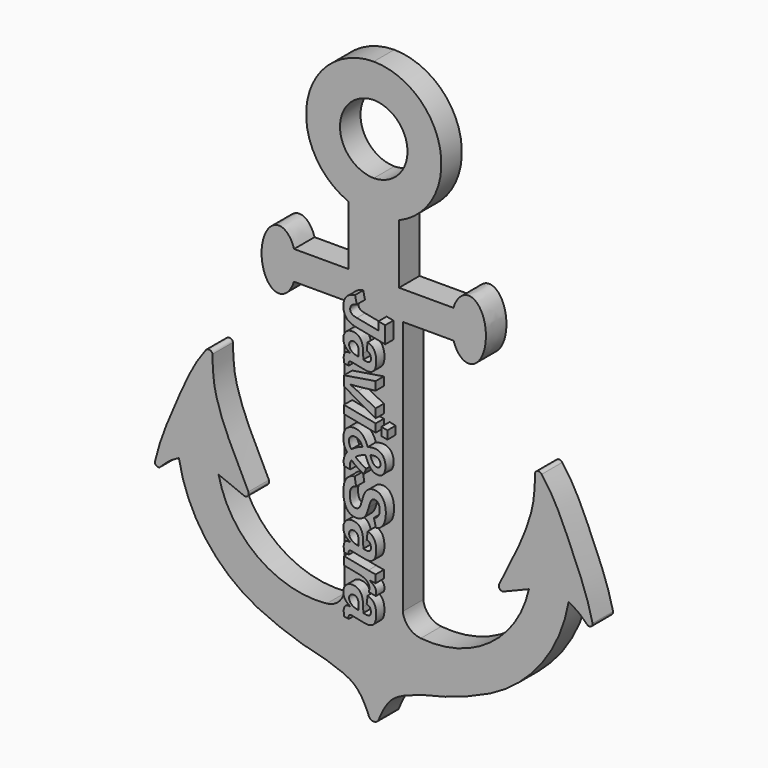
from build123d import *

# Parameters (mm, degrees)
F1_DEPTH     = 2.5
F2_TEXT_SIZE = 5.843307762
F3_DEPTH     = 1


# Not quite as in the source:
# - Text() gives the source's letters only with a copy of the font that has no kerning and outlines rounded to 1/6400 em; it was checked with that copy


with BuildPart() as f1:
    # F0 (on Front) → F1 (new body)
    with BuildSketch(Plane.XZ):
        Polygon((19.9702170016, 32.0593795983), (15.0368500231, 32.0593795983), (15.0368500231, 26.2546902991), (9.737966444, 26.2546902991), (9.7163520504, 23.4430860728), (14.649162069, 23.4430860728), (14.649162069, -1.4119866537), (14.6655309945, -1.4119866537), (20.3415360302, -1.4119866537), (20.3579049557, -1.4119866537), (20.3579049557, 23.4430860728), (25.2907149743, 23.4430860728), (25.2767818304, 26.2546902991), (25.2691005807, 26.2546902991), (19.9702170016, 26.2546902991), align=None)
        with BuildLine():
            add(Edge.make_bspline(
                [(25.2907149743, 23.4430860728), (26.2882305831, 20.365262945), (27.8484616427, 22.637675937), (29.4086927023, 24.9100889291), (27.8261704411, 27.1358736943), (26.2436481799, 29.3616584594), (25.2767818304, 26.2546902991)],
                knots=[2.0818835057, 2.0818835057, 2.0818835057, 3.8412701203, 3.8412701203, 5.6006567348, 5.6006567348, 7.3600433494, 7.3600433494, 7.3600433494], degree=2, weights=[1, 0.6373874942, 1, 0.6373874942, 1, 0.6373874942, 1]))
            Line((25.2767818304, 26.2546902991), (25.2907149743, 23.4430860728))
        make_face()
        with BuildLine():
            ThreePointArc((19.9702170016, 32.0593795983), (23.9805343506, 39.4793828594), (17.5035335124, 44.8819335324))
            ThreePointArc((17.5035335124, 44.8819335324), (11.0265326741, 39.4793828594), (15.0368500231, 32.0593795983))
            Line((15.0368500231, 32.0593795983), (19.9702170016, 32.0593795983))
        make_face()
        with BuildLine():
            ThreePointArc((17.5035335124, 34.864031021), (14.2101902268, 38.22103329), (17.5035335124, 41.578035559))
            ThreePointArc((17.5035335124, 41.578035559), (20.796876798, 38.22103329), (17.5035335124, 34.864031021))
        make_face(mode=Mode.SUBTRACT)
        with BuildLine():
            Line((9.7163520504, 23.4430860728), (9.737966444, 26.2546902991))
            Line((9.737966444, 26.2546902991), (9.7302851943, 26.2546902991))
            add(Edge.make_bspline(
                [(9.7302851943, 26.2546902991), (8.7634188448, 29.3616584594), (7.1808965836, 27.1358736943), (5.5983743224, 24.9100889291), (7.158605382, 22.637675937), (8.7188364416, 20.365262945), (9.7163520504, 23.4430860728)],
                knots=[5.206327265, 5.206327265, 5.206327265, 6.9657138795, 6.9657138795, 8.7251004941, 8.7251004941, 10.4844871087, 10.4844871087, 10.4844871087], degree=2, weights=[1, 0.6373874942, 1, 0.6373874942, 1, 0.6373874942, 1]))
        make_face()
        with BuildLine():
            Line((20.3415360302, -1.4119866537), (14.6655309945, -1.4119866537))
            ThreePointArc((14.6655309945, -1.4119866537), (14.104262397, -2.601770472), (12.9159725396, -3.1661951243))
            ThreePointArc((12.9159725396, -3.1661951243), (6.1837849457, -1.3494681757), (2.3638433989, 4.4841321865))
            Line((2.3638433989, 4.4841321865), (-1.5069706133, 4.6396357939))
            ThreePointArc((-1.5069706133, 4.6396357939), (1.0924430649, -1.4370902061), (6.1424945269, -5.7009535458))
            ThreePointArc((6.1424945269, -5.7009535458), (9.411755425, -7.0527797683), (12.8207588568, -7.9983994365))
            add(Edge.make_bspline(
                [(12.8207588568, -7.9983994365), (13.2286113889, -8.1298598572), (14.030525637, -8.3883355957), (15.1474289659, -8.8652634772), (16.0285297181, -9.5488398221), (16.7051850381, -10.7003064264), (16.9278864722, -11.2527367175), (17.0273277909, -11.4994095638)],
                knots=[0, 0, 0, 0, 0.2115418785, 0.4159308405, 0.6130256954, 0.8272070618, 1, 1, 1, 1], degree=3))
            ThreePointArc((17.0273277909, -11.4994095638), (17.2146874841, -11.731113087), (17.5035335124, -11.8043124676))
            ThreePointArc((17.5035335124, -11.8043124676), (17.7923795406, -11.731113087), (17.9797392339, -11.4994095638))
            add(Edge.make_bspline(
                [(22.1863081679, -7.9983994365), (21.7784556358, -8.1298598572), (20.9765413877, -8.3883355957), (19.8596380588, -8.8652634772), (18.9785373066, -9.5488398221), (18.3018819866, -10.7003064264), (18.0791805525, -11.2527367175), (17.9797392339, -11.4994095638)],
                knots=[0, 0, 0, 0, 0.2115418785, 0.4159308405, 0.6130256954, 0.8272070618, 1, 1, 1, 1], degree=3))
            ThreePointArc((22.1863081679, -7.9983994365), (25.5953115998, -7.0527797683), (28.8645724978, -5.7009535458))
            ThreePointArc((28.8645724978, -5.7009535458), (33.9146239598, -1.4370902061), (36.514037638, 4.6396357939))
            Line((36.514037638, 4.6396357939), (32.6432236258, 4.4841321865))
            ThreePointArc((32.6432236258, 4.4841321865), (28.823282079, -1.3494681757), (22.0910944851, -3.1661951243))
            ThreePointArc((22.0910944851, -3.1661951243), (20.9028046278, -2.601770472), (20.3415360302, -1.4119866537))
        make_face()
        with BuildLine():
            Line((-1.5069706133, 4.6396357939), (2.3638433989, 4.4841321865))
            Line((2.3638433989, 4.4841321865), (4.8265583094, 3.4840409858))
            ThreePointArc((4.8265583094, 3.4840409858), (5.207101451, 3.5650237911), (5.2730236415, 3.9484629156))
            add(Edge.make_bspline(
                [(5.2730236415, 3.9484629156), (4.3093190608, 5.8568781898), (2.6415257191, 9.1595939302), (1.7918217485, 12.3374978629), (1.7806474113, 13.9165389117), (1.7755767331, 14.6330744028)],
                knots=[0, 0, 0, 0, 0.4277955284, 0.7403456912, 1, 1, 1, 1], degree=3))
            ThreePointArc((1.7755767331, 14.6330744028), (1.4853684877, 14.9141883565), (1.1110873893, 14.7620057687))
            add(Edge.make_bspline(
                [(1.1110873893, 14.7620057687), (0, 13.3479235297), (-1.5371329646, 9.9603936039), (-3.3933382019, 5.6264709941), (-3.8495825403, 3.5681225897)],
                knots=[0, 0, 0, 0, 0.4745849169, 1, 1, 1, 1], degree=3))
            ThreePointArc((-3.8495825403, 3.5681225897), (-3.713409423, 3.2620784428), (-3.3794315532, 3.2362923957))
            add(Edge.make_bspline(
                [(-3.3794315532, 3.2362923957), (-3.0844818323, 3.5324643819), (-2.5082629775, 4.1110710752), (-1.8354097748, 4.4662585074), (-1.5069706133, 4.6396357939)],
                knots=[0, 0, 0, 0, 0.5118709991, 1, 1, 1, 1], degree=3))
        make_face()
        with BuildLine():
            Line((30.1805087153, 3.4840409858), (32.6432236258, 4.4841321865))
            Line((32.6432236258, 4.4841321865), (36.514037638, 4.6396357939))
            add(Edge.make_bspline(
                [(38.3864985779, 3.2362923957), (38.091548857, 3.5324643819), (37.5153300022, 4.1110710752), (36.8424767996, 4.4662585074), (36.514037638, 4.6396357939)],
                knots=[0, 0, 0, 0, 0.5118709991, 1, 1, 1, 1], degree=3))
            ThreePointArc((38.3864985779, 3.2362923957), (38.7204764477, 3.2620784428), (38.856649565, 3.5681225897))
            add(Edge.make_bspline(
                [(33.8959796354, 14.7620057687), (35.0070670247, 13.3479235297), (36.5441999893, 9.9603936039), (38.4004052267, 5.6264709941), (38.856649565, 3.5681225897)],
                knots=[0, 0, 0, 0, 0.4745849169, 1, 1, 1, 1], degree=3))
            ThreePointArc((33.8959796354, 14.7620057687), (33.521698537, 14.9141883565), (33.2314902917, 14.6330744028))
            add(Edge.make_bspline(
                [(29.7340433832, 3.9484629156), (30.6977479639, 5.8568781898), (32.3655413056, 9.1595939302), (33.2152452762, 12.3374978629), (33.2264196134, 13.9165389117), (33.2314902917, 14.6330744028)],
                knots=[0, 0, 0, 0, 0.4277955284, 0.7403456912, 1, 1, 1, 1], degree=3))
            ThreePointArc((29.7340433832, 3.9484629156), (29.7999655737, 3.5650237911), (30.1805087153, 3.4840409858))
        make_face()
    extrude(amount=F1_DEPTH)

    # F2 (on face) → F3 (join)
    with BuildSketch(Plane.XZ.offset(2.5)):
        with Locations(Location((15.3999431059, 24.9723309247), (0, 0, -90))):
            Text('Javi&Sara', F2_TEXT_SIZE, font='Arimo', font_style=FontStyle.BOLDITALIC, text_align=(TextAlign.LEFT, TextAlign.BOTTOM))
    extrude(amount=F3_DEPTH)


solid = f1.part
